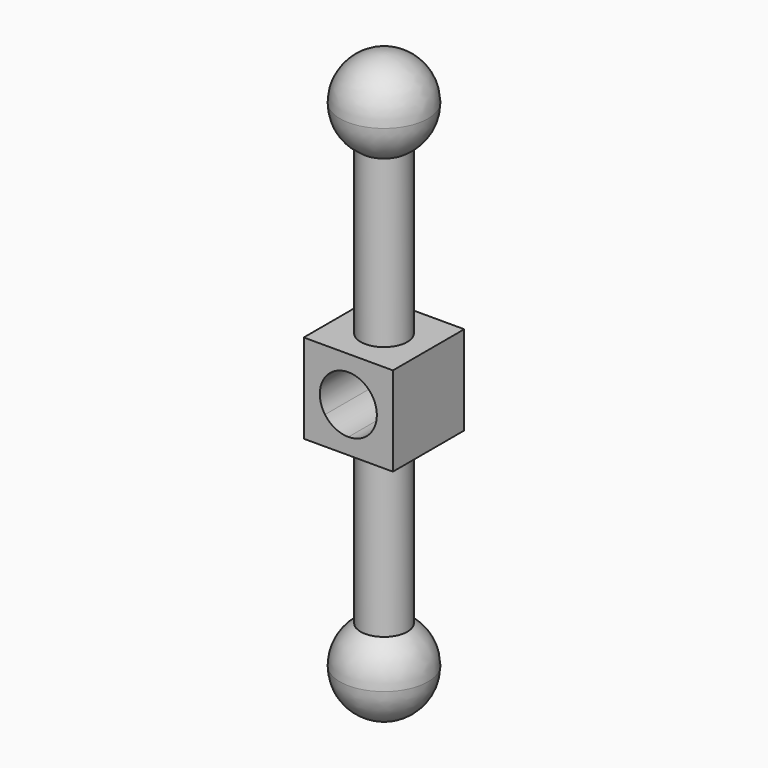
from build123d import *

# Parameters (mm, degrees)
F1_DEPTH = 12.5


with BuildPart() as f1:
    # F0 (on Front) → F1 (new body, symmetric)
    with BuildSketch(Plane.XZ):
        with BuildLine():
            Line((-12.5, -12.5), (-6.541519, -12.5))
            Line((-6.541519, -12.5), (-6.541519, -4.605271))
            ThreePointArc((-6.541519, -4.605271), (-8, 0), (-6.541519, 4.605271))
            Line((-6.541519, 4.605271), (-6.541519, 12.5))
            Line((-6.541519, 12.5), (-12.5, 12.5))
            Line((-12.5, 12.5), (-12.5, -12.5))
        make_face()
        with BuildLine():
            Line((6.541519, -4.605271), (6.541519, -12.5))
            Line((6.541519, -12.5), (12.5, -12.5))
            Line((12.5, -12.5), (12.5, 12.5))
            Line((12.5, 12.5), (6.541519, 12.5))
            Line((6.541519, 12.5), (6.541519, 4.605271))
            ThreePointArc((6.541519, 4.605271), (7.626669, 2.415351), (8, 0))
            ThreePointArc((8, 0), (7.626669, -2.415351), (6.541519, -4.605271))
        make_face()
        with BuildLine():
            Line((-6.541519, 12.5), (-6.541519, 4.605271))
            ThreePointArc((-6.541519, 4.605271), (-3.684958, 7.100781), (0, 8))
            Line((0, 8), (0, 12.5))
            Line((0, 12.5), (-6.541519, 12.5))
        make_face()
        with BuildLine():
            Line((-6.541519, -4.605271), (-6.541519, -12.5))
            Line((-6.541519, -12.5), (0, -12.5))
            Line((0, -12.5), (0, -8))
            ThreePointArc((0, -8), (-3.684958, -7.100781), (-6.541519, -4.605271))
        make_face()
        with BuildLine():
            Line((0, 12.5), (0, 8))
            ThreePointArc((0, 8), (3.684958, 7.100781), (6.541519, 4.605271))
            Line((6.541519, 4.605271), (6.541519, 12.5))
            Line((6.541519, 12.5), (0, 12.5))
        make_face()
        with BuildLine():
            Line((0, -8), (0, -12.5))
            Line((0, -12.5), (6.541519, -12.5))
            Line((6.541519, -12.5), (6.541519, -4.605271))
            ThreePointArc((6.541519, -4.605271), (3.684958, -7.100781), (0, -8))
        make_face()
    extrude(amount=F1_DEPTH, both=True)


with BuildPart() as f2:
    # F0 (on Front) → F2 (revolve)
    with BuildSketch(Plane.XZ):
        with BuildLine():
            Line((0, 57.161123), (0, 12.5))
            Line((0, 12.5), (6.541519, 12.5))
            Line((6.541519, 12.5), (6.541519, 59.037207))
            ThreePointArc((6.541519, 59.037207), (3.402615, 57.639411), (0, 57.161123))
        make_face()
    revolve(axis=Axis((0, 0, 0), (0, 0, -1)))


with BuildPart() as f2b:
    # F0 (on Front) → F2, piece 2 (revolve)
    with BuildSketch(Plane.XZ):
        with BuildLine():
            Line((0, -12.5), (0, -57.161123))
            ThreePointArc((0, -57.161123), (3.402615, -57.639411), (6.541519, -59.037207))
            Line((6.541519, -59.037207), (6.541519, -12.5))
            Line((6.541519, -12.5), (0, -12.5))
        make_face()
    revolve(axis=Axis((0, 0, 0), (0, 0, -1)))


with BuildPart() as f3:
    # F0 (on Front) → F3 (revolve)
    with BuildSketch(Plane.XZ):
        with BuildLine():
            ThreePointArc((12.342512, 69.503635), (8.727474, 78.231109), (0, 81.846147))
            Line((0, 81.846147), (0, 69.503635))
            Line((0, 69.503635), (6.541519, 69.503635))
            Line((6.541519, 69.503635), (6.541519, 59.037207))
            ThreePointArc((6.541519, 59.037207), (10.795286, 63.520375), (12.342512, 69.503635))
        make_face()
    revolve(axis=Axis((0, 0, 75.674891), (0, 0, 1)))


with BuildPart() as f3b:
    # F0 (on Front) → F3, piece 2 (revolve)
    with BuildSketch(Plane.XZ):
        with BuildLine():
            Line((6.541519, -69.503635), (0, -69.503635))
            Line((0, -69.503635), (0, -81.846147))
            ThreePointArc((0, -81.846147), (8.727474, -78.231109), (12.342512, -69.503635))
            ThreePointArc((12.342512, -69.503635), (10.795286, -63.520375), (6.541519, -59.037207))
            Line((6.541519, -59.037207), (6.541519, -69.503635))
        make_face()
    revolve(axis=Axis((0, 0, 75.674891), (0, 0, 1)))


with BuildPart() as f1_1:
    add(f1.part)

    # F4: union F2, F2b, F3, F3b
    add(f2.part)
    add(f2b.part)
    add(f3.part)
    add(f3b.part)


solid = f1_1.part
